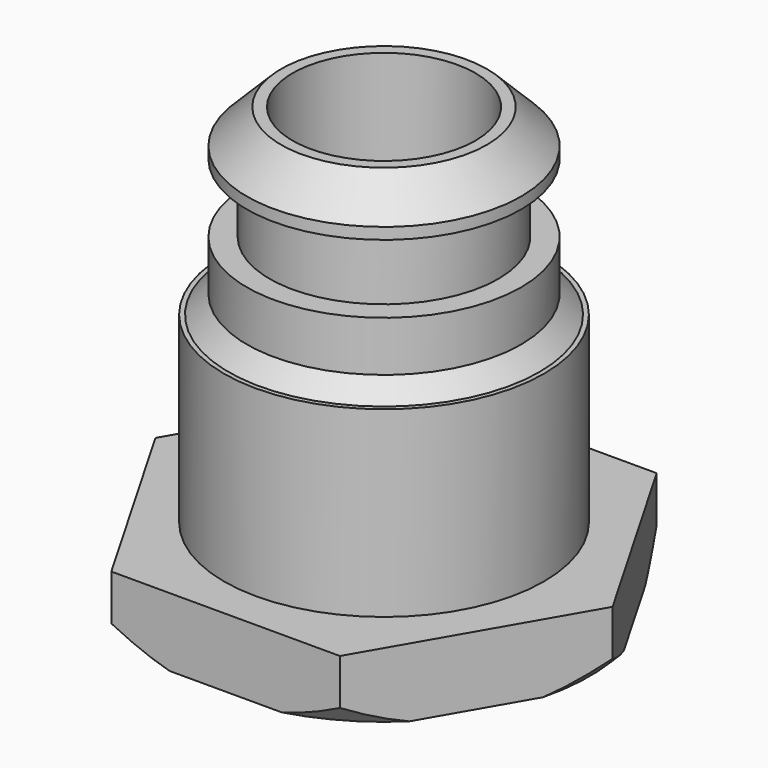
from build123d import *

# Parameters (mm, degrees)
F2_SIZE      = 2.54
F4_DEPTH     = 60.326
F5_SIZE      = 4.7625
F6_TEXT_SIZE = 0.9852784197
F7_DEPTH     = 25.4


# Not quite as in the source:
# - Text() gives the source's letters only with a copy of the font that has no kerning and outlines rounded to 1/6400 em; it was checked with that copy


with BuildPart() as f1:
    # F0 (on Front) → F1 (revolve)
    with BuildSketch(Plane.XZ):
        Polygon((12.7, 60.325), (12.7, 0), (28.575, 0), (31.75, 3.175), (31.75, 9.525), (22.225, 9.525), (22.225, 34.925), (19.05, 34.925), (19.05, 44.45), (15.875, 44.45), (15.875, 53.975), (19.05, 53.975), (19.05, 60.325), align=None)
    revolve(axis=Axis((0, 0, 30.1625), (0, 0, 1)))

    # F2
    f2_edges = [f1.edges().sort_by_distance(p)[0] for p in [
        (-19.05, 0, 34.925),
    ]]
    chamfer(f2_edges, length=F2_SIZE)

    # F3 (on Top) → F4 (cut, through all)
    with BuildSketch(Plane.XY):
        with BuildLine():
            Line((-15.875, -27.4963065702), (-31.75, 0))
            ThreePointArc((-31.75, 0), (-27.4963065702, -15.875), (-15.875, -27.4963065702))
        make_face()
        with BuildLine():
            Line((-31.75, 0), (-15.875, 27.4963065702))
            ThreePointArc((-15.875, 27.4963065702), (-27.4963065702, 15.875), (-31.75, 0))
        make_face()
        with BuildLine():
            Line((-15.875, 27.4963065702), (15.875, 27.4963065702))
            ThreePointArc((15.875, 27.4963065702), (0, 31.75), (-15.875, 27.4963065702))
        make_face()
        with BuildLine():
            ThreePointArc((31.75, 0), (27.4963065702, 15.875), (15.875, 27.4963065702))
            Line((15.875, 27.4963065702), (31.75, 0))
        make_face()
        with BuildLine():
            ThreePointArc((15.875, -27.4963065702), (27.4963065702, -15.875), (31.75, 0))
            Line((31.75, 0), (15.875, -27.4963065702))
        make_face()
        with BuildLine():
            ThreePointArc((-15.875, -27.4963065702), (0, -31.75), (15.875, -27.4963065702))
            Line((15.875, -27.4963065702), (-15.875, -27.4963065702))
        make_face()
    extrude(amount=F4_DEPTH, mode=Mode.SUBTRACT)

    # F5
    f5_edges = [f1.edges().sort_by_distance(p)[0] for p in [
        (-19.05, 0, 60.325),
    ]]
    chamfer(f5_edges, length=F5_SIZE)

    # F6 (on face) → F7 (cut)
    with BuildSketch(Plane(origin=(0, 0, 0), x_dir=(1, 0, 0), z_dir=(0, 0, -1))):
        with Locations((-19.0248112376, 5.2083478076)):
            Text('Mobile App Test', F6_TEXT_SIZE, font='Open Sans', text_align=(TextAlign.LEFT, TextAlign.BOTTOM))
    extrude(amount=-F7_DEPTH, mode=Mode.SUBTRACT)


solid = f1.part
